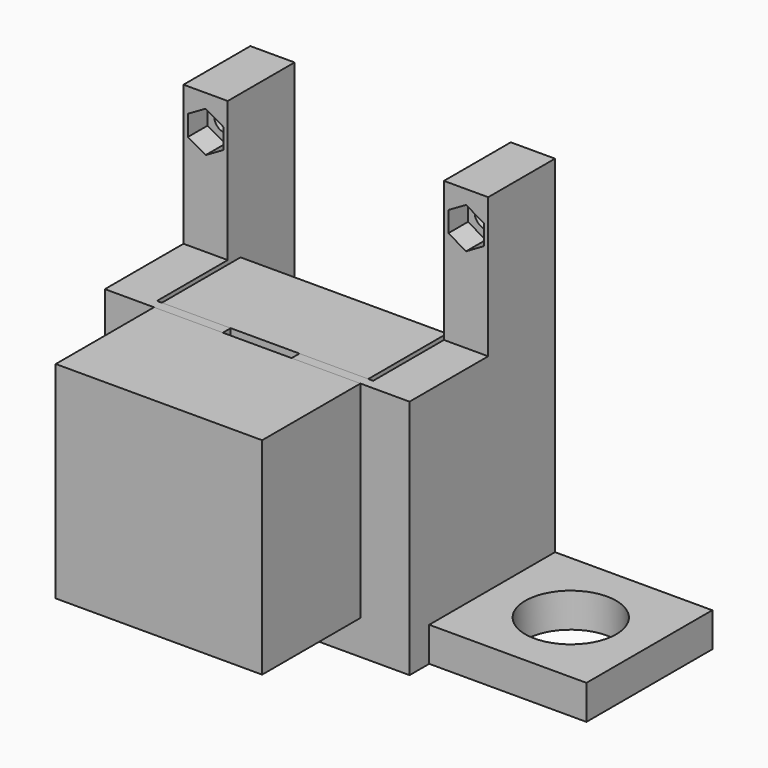
from build123d import *

# Parameters (mm, degrees)
F1_R      = 2.25
F2_DEPTH  = 12
F4_DEPTH  = 5
F5_W      = 44
F5_H      = 18
F5_H_2    = 2
F6_DEPTH  = 7
F7_DEPTH  = 42
F8_R      = 1.7
F8_R_2    = 13
F9_DEPTH  = 2
F11_REACH = 63.1431356237
F12_R     = 1.7
F13_DEPTH = 20
F14_W     = 42
F14_H     = 42
F14_R     = 1.7
F14_R_2   = 13
F15_DEPTH = 25
F16_W     = 32
F16_H     = 32
F16_R     = 9.25
F17_DEPTH = 7
F18_W     = 44
F18_H     = 23.4653228298
F18_R     = 2.25
F19_DEPTH = 5
F20_R     = 2.25
F21_DEPTH = 3


with BuildPart() as f2:
    # F1 (on Front) → F2 (new body)
    with BuildSketch(Plane.XZ):
        Polygon((-27, 56.5), (-36, 56.5), (-36, -21), (26, -21), (26, 56.5), (17, 56.5), (17, -14), (-27, -14), align=None)
        with Locations((-31.5, 49.5)):
            Circle(F1_R, mode=Mode.SUBTRACT)
        with Locations((21.5, 49.5)):
            Circle(F1_R, mode=Mode.SUBTRACT)
    extrude(amount=-F2_DEPTH)

    # F3 (on face) → F4 (join)
    with BuildSketch(Plane.XZ):
        Polygon((-27, -14), (-27, 56.5), (-36, 56.5), (-36, -21), (26, -21), (26, 56.5), (17, 56.5), (17, -14), align=None)
        Polygon((-31.5, 53.6569219382), (-27.9, 51.5784609691), (-27.9, 47.4215390309), (-31.5, 45.3430780618), (-35.1, 47.4215390309), (-35.1, 51.5784609691), align=None, mode=Mode.SUBTRACT)
        Polygon((21.5, 53.6569219382), (25.1, 51.5784609691), (25.1, 47.4215390309), (21.5, 45.3430780618), (17.9, 47.4215390309), (17.9, 51.5784609691), align=None, mode=Mode.SUBTRACT)
    extrude(amount=F4_DEPTH)

    # F5 (on face) → F6 (join, through all)
    with BuildSketch(Plane.XY.offset(-14)):
        with Locations((-5, -14)):
            Rectangle(F5_W, F5_H)
        with Locations((-5, -24)):
            Rectangle(F5_W, F5_H_2)
        Polygon((-27, -23), (-27, -5), (-36, -5), (-36, -25), (-27, -25), align=None)
        Polygon((26, -5), (17, -5), (17, -23), (17, -25), (26, -25), align=None)
    extrude(amount=-F6_DEPTH)

    # F5 (on face) → F7 (join)
    with BuildSketch(Plane.XY.offset(-14)):
        with Locations((-5, -24)):
            Rectangle(F5_W, F5_H_2)
        Polygon((-27, -23), (-27, -5), (-36, -5), (-36, -25), (-27, -25), align=None)
        Polygon((26, -5), (17, -5), (17, -23), (17, -25), (26, -25), align=None)
    extrude(amount=F7_DEPTH)

    # F8 (on face) → F9 (cut, through all)
    with BuildSketch(Plane.XZ.offset(25)):
        with Locations((-20.5, 22.5)):
            Circle(F8_R)
        with Locations((-5, 7)):
            Circle(F8_R_2)
        with Locations((-20.5, -8.5)):
            Circle(F8_R)
        with Locations((10.5, -8.5)):
            Circle(F8_R)
        with Locations((10.5, 22.5)):
            Circle(F8_R)
    extrude(amount=-F9_DEPTH, mode=Mode.SUBTRACT)

    f11_end = f2.faces().sort_by_distance((-18, -24, 7))[0]
    # F10 (on face) → F11 (cut, up to a face of the model that its end follows)
    with BuildSketch(Plane.XY.offset(28)):
        Polygon((2, -23), (-5, -23), (-12, -23), (-12, -25), (2, -25), align=None)
    f11_long = extrude(amount=-F11_REACH, mode=Mode.PRIVATE)
    add(split(f11_long, bisect_by=f11_end, keep=Keep.ALL, mode=Mode.PRIVATE).solids().sort_by_distance((-5, -24, 28))[0], mode=Mode.SUBTRACT)

    # F18 (on face) → F19 (join)
    with BuildSketch(Plane(origin=(0, 12, 0), x_dir=(-1, 0, 0), z_dir=(0, 1, 0))):
        with Locations((5, -2.2673385851)):
            Rectangle(F18_W, F18_H)
        Circle(F18_R, mode=Mode.SUBTRACT)
    extrude(amount=-F19_DEPTH)

    # F20 (on face) → F21 (cut)
    with BuildSketch(Plane.XZ.offset(-7)):
        Polygon((-0.410156085, 4.2290001548), (-3.8674996092, 1.7592944883), (-3.4573435242, -2.4697056666), (0.410156085, -4.2290001548), (3.8674996092, -1.7592944883), (3.4573435242, 2.4697056666), align=None)
        Circle(F20_R, mode=Mode.SUBTRACT)
    extrude(amount=-F21_DEPTH, mode=Mode.SUBTRACT)


with BuildPart() as f13:
    # F12 (on face) → F13 (new body)
    with BuildSketch(Plane(origin=(0, -23, 0), x_dir=(-1, 0, 0), z_dir=(0, 1, 0))):
        with BuildLine():
            Line((-16, -14), (26, -14))
            Line((26, -14), (26, 28))
            Line((26, 28), (12, 28))
            Line((12, 28), (12, 17.9544511501))
            ThreePointArc((12, 17.9544511501), (5, -6), (-2, 17.9544511501))
            Line((-2, 17.9544511501), (-2, 28))
            Line((-2, 28), (-16, 28))
            Line((-16, 28), (-16, -14))
        make_face()
        with Locations((-10.5, -8.5)):
            Circle(F12_R, mode=Mode.SUBTRACT)
        with Locations((20.5, -8.5)):
            Circle(F12_R, mode=Mode.SUBTRACT)
        with Locations((-10.5, 22.5)):
            Circle(F12_R, mode=Mode.SUBTRACT)
        with Locations((20.5, 22.5)):
            Circle(F12_R, mode=Mode.SUBTRACT)
        with BuildLine():
            Line((12, 17.9544511501), (12, 28))
            Line((12, 28), (-2, 28))
            Line((-2, 28), (-2, 17.9544511501))
            ThreePointArc((-2, 17.9544511501), (5, -6), (12, 17.9544511501))
        make_face()
        with Locations((-10.5, 22.5)):
            Circle(F12_R)
        with Locations((20.5, 22.5)):
            Circle(F12_R)
        with Locations((-10.5, -8.5)):
            Circle(F12_R)
        with Locations((20.5, -8.5)):
            Circle(F12_R)
    extrude(amount=F13_DEPTH)


with BuildPart() as f15:
    # F14 (on face) → F15 (new body)
    with BuildSketch(Plane.XZ.offset(25)):
        with Locations((-5, 7)):
            Rectangle(F14_W, F14_H)
        with Locations((-20.5, -8.5)):
            Circle(F14_R, mode=Mode.SUBTRACT)
        with Locations((10.5, -8.5)):
            Circle(F14_R, mode=Mode.SUBTRACT)
        with Locations((-20.5, 22.5)):
            Circle(F14_R, mode=Mode.SUBTRACT)
        with Locations((-5, 7)):
            Circle(F14_R_2, mode=Mode.SUBTRACT)
        with Locations((10.5, 22.5)):
            Circle(F14_R, mode=Mode.SUBTRACT)
    extrude(amount=F15_DEPTH)

    # F8 (on face) → F15, piece 2 (join)
    with BuildSketch(Plane.XZ.offset(25)):
        with Locations((-20.5, 22.5)):
            Circle(F8_R)
    extrude(amount=F15_DEPTH)

    # F8 (on face) → F15, piece 3 (join)
    with BuildSketch(Plane.XZ.offset(25)):
        with Locations((-5, 7)):
            Circle(F8_R_2)
    extrude(amount=F15_DEPTH)

    # F8 (on face) → F15, piece 4 (join)
    with BuildSketch(Plane.XZ.offset(25)):
        with Locations((-20.5, -8.5)):
            Circle(F8_R)
    extrude(amount=F15_DEPTH)

    # F8 (on face) → F15, piece 5 (join)
    with BuildSketch(Plane.XZ.offset(25)):
        with Locations((10.5, 22.5)):
            Circle(F8_R)
    extrude(amount=F15_DEPTH)

    # F8 (on face) → F15, piece 6 (join)
    with BuildSketch(Plane.XZ.offset(25)):
        with Locations((10.5, -8.5)):
            Circle(F8_R)
    extrude(amount=F15_DEPTH)


with BuildPart() as f17:
    # F16 (on face) → F17 (new body, through all)
    with BuildSketch(Plane(origin=(0, 0, -21), x_dir=(1, 0, 0), z_dir=(0, 0, -1))):
        with Locations((42, 4)):
            Rectangle(F16_W, F16_H)
        with Locations((42, 4)):
            Circle(F16_R, mode=Mode.SUBTRACT)
    extrude(amount=-F17_DEPTH)


solid = Compound([f2.part, f13.part, f15.part, f17.part])
